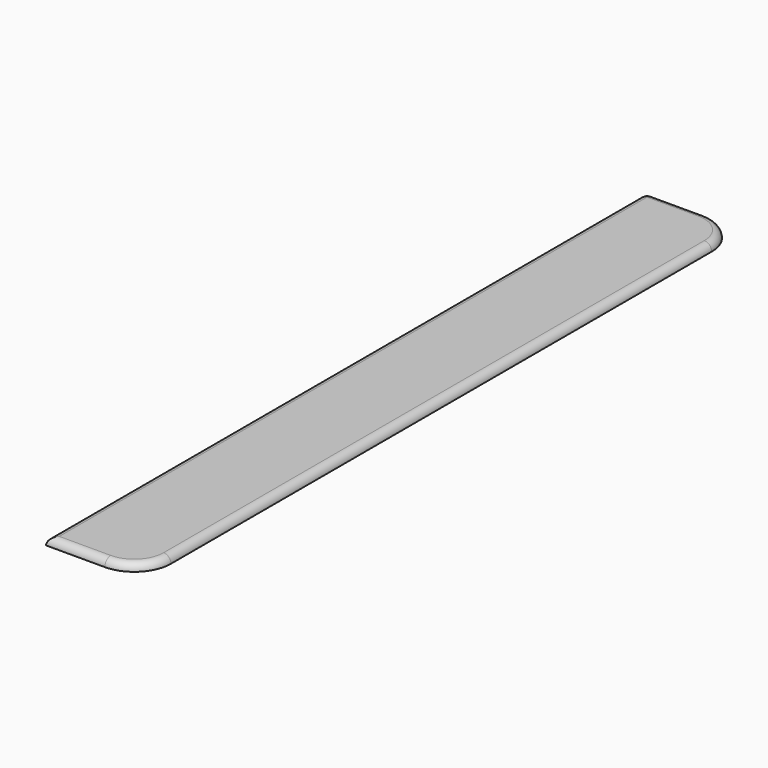
from build123d import *

# Parameters (mm, degrees)
F1_DEPTH     = 1
F2_W         = 1.7
F2_H         = 2
F2_W_2       = 6.3
F2_H_2       = 8
F3_DEPTH     = 1.7
F4_W         = 8
F4_H         = 10
F5_DEPTH     = 2
F6_R         = 5
F7_R         = 0.99999
F8_T1_DEPTH  = 3.7
F8_T3_DEPTH  = 7.5
F8_T5_DEPTH  = 9.5
F8_T7_DEPTH  = 5.5
F8_T9_DEPTH  = 11.5
F8_T12_ANGLE = 90
F8_S15_W     = 1
F8_S15_H     = 1
F8_T16_DEPTH = 1
F8_T20_ANGLE = 90
F10_DEPTH    = 1.7


# Not quite as in the source:
# - a fillet or chamfer that OpenCascade refuses, or shapes differently, is made with other operations: its cross-section is extruded or revolved along the edge and cut away or added
# - a fillet or chamfer is up to 0.001 mm smaller than in the source, because OpenCascade refuses the exact size


with BuildPart() as f1:
    # F0 (on Top) → F1 (new body)
    with BuildSketch(Plane.XY):
        with BuildLine():
            Line((-6.5, -51), (6.5, -51))
            Line((6.5, -51), (6.5, 46))
            ThreePointArc((6.5, 46), (5.0355339059, 49.5355339059), (1.5, 51))
            Line((1.5, 51), (-6.5, 51))
            Line((-6.5, 51), (-6.5, -51))
        make_face()
    extrude(amount=F1_DEPTH)

    # F2 (on face) → F3 (join)
    with BuildSketch(Plane(origin=(0, 0, 0), x_dir=(1, 0, 0), z_dir=(0, 0, -1))):
        with Locations((-5.65, -50)):
            Rectangle(F2_W, F2_H)
        with Locations((-1.65, -50)):
            Rectangle(F2_W_2, F2_H)
        with Locations((-5.65, -45)):
            Rectangle(F2_W, F2_H_2)
    extrude(amount=F3_DEPTH)

    # F4 (on face) → F5 (join)
    with BuildSketch(Plane(origin=(0, 0, -1.7), x_dir=(1, 0, 0), z_dir=(0, 0, -1))):
        with Locations((-2.5, -46)):
            Rectangle(F4_W, F4_H)
    extrude(amount=F5_DEPTH)

    # F6
    f6_edges = [f1.edges().sort_by_distance(p)[0] for p in [
        (6.5, -51, 0.5),
        (1.5, 41, -2.7),
    ]]
    fillet(f6_edges, radius=F6_R)

    # F7 (radius 1 in the source; OpenCascade refuses exactly that, so slightly less here)
    f7_edges = [f1.edges().sort_by_distance(p)[0] for p in [
        (-2.5, -51, 1),
        (5.035534, -49.535534, 1),
        (-6.5, 0, 1),
        (6.5, 0, 1),
        (-2.5, 51, 1),
        (5.035534, 49.535534, 1),
    ]]
    fillet(f7_edges, radius=F7_R)

    # F8: fillet of radius 1 on 6 edges, made by hand

    # F8_s2 → F8_t1 (cut)
    with BuildSketch(Plane.XY.offset(-2.7)):
        with BuildLine():
            ThreePointArc((-5.5, 51), (-6.2071067812, 50.7071067812), (-6.5, 50))
            Line((-6.5, 50), (-6.5, 51))
            Line((-6.5, 51), (-5.5, 51))
        make_face()
    extrude(amount=F8_T1_DEPTH, mode=Mode.SUBTRACT)

    # F8_s4 → F8_t3 (cut)
    with BuildSketch(Plane.XZ.offset(-53.5)):
        with BuildLine():
            ThreePointArc((1.5, -2.7), (1.2071067812, -3.4071067812), (0.5, -3.7))
            Line((0.5, -3.7), (1.5, -3.7))
            Line((1.5, -3.7), (1.5, -2.7))
        make_face()
    extrude(amount=F8_T3_DEPTH, mode=Mode.SUBTRACT)

    # F8_s6 → F8_t5 (cut)
    with BuildSketch(Plane.YZ.offset(-5.5)):
        with BuildLine():
            ThreePointArc((51, -2.7), (50.7071067812, -3.4071067812), (50, -3.7))
            Line((50, -3.7), (51, -3.7))
            Line((51, -3.7), (51, -2.7))
        make_face()
    extrude(amount=F8_T5_DEPTH, mode=Mode.SUBTRACT)

    # F8_s8 → F8_t7 (cut)
    with BuildSketch(Plane.YZ.offset(-9)):
        with BuildLine():
            ThreePointArc((42, -3.7), (41.2928932188, -3.4071067812), (41, -2.7))
            Line((41, -2.7), (41, -3.7))
            Line((41, -3.7), (42, -3.7))
        make_face()
    extrude(amount=F8_T7_DEPTH, mode=Mode.SUBTRACT)

    # F8_s10 → F8_t9 (cut)
    with BuildSketch(Plane.XZ.offset(-50)):
        with BuildLine():
            ThreePointArc((-6.5, -2.7), (-6.2071067812, -3.4071067812), (-5.5, -3.7))
            Line((-5.5, -3.7), (-6.5, -3.7))
            Line((-6.5, -3.7), (-6.5, -2.7))
        make_face()
    extrude(amount=F8_T9_DEPTH, mode=Mode.SUBTRACT)

    # F8_s11 → F8_t12 (revolve, cut)
    with BuildSketch(Plane.YZ.offset(-5.5)):
        with BuildLine():
            ThreePointArc((50.00001, 1), (50.7071097101, 0.7071097101), (51, 1e-05))
            Line((51, 1e-05), (51, 1))
            Line((51, 1), (50.00001, 1))
        make_face()
    revolve(axis=Axis((-5.5, 50, 1), (0, 0, 1)), revolution_arc=F8_T12_ANGLE, mode=Mode.SUBTRACT)


with BuildPart() as f8_tool14:
    # F8_s15 → F8_t16 (new body)
    with BuildSketch(Plane.XZ.offset(-50)):
        with Locations((-6, -3.2)):
            Rectangle(F8_S15_W, F8_S15_H)
    extrude(amount=-F8_T16_DEPTH)

    # F8_s17 → F8_t18 (revolve, cut)
    with BuildSketch(Plane(origin=(-5.5, 50, -2.7), x_dir=(0.7071067812, 0, 0.7071067812), z_dir=(-0.7071067812, 0, 0.7071067812))):
        with BuildLine():
            ThreePointArc((0, -1), (1, 0), (0, 1))
            Line((0, 1), (0, -1))
        make_face()
    revolve(axis=Axis((-5.5, 50, -2.7), (0, 1, 0)), mode=Mode.SUBTRACT)


with BuildPart() as f1_1:
    add(f1.part)

    # F8_t13: cut F8_tool14
    add(f8_tool14.part, mode=Mode.SUBTRACT)

    # F8_s19 → F8_t20 (revolve, cut)
    with BuildSketch(Plane.XZ.offset(-46)):
        with BuildLine():
            ThreePointArc((0.5, -3.7), (1.2071067812, -3.4071067812), (1.5, -2.7))
            Line((1.5, -2.7), (1.5, -3.7))
            Line((1.5, -3.7), (0.5, -3.7))
        make_face()
    revolve(axis=Axis((-3.5, 46, -3.7), (0, 0, -1)), revolution_arc=F8_T20_ANGLE, mode=Mode.SUBTRACT)

    # F9 (on face) → F10 (join, through all)
    with BuildSketch(Plane(origin=(0, 0, 0), x_dir=(1, 0, 0), z_dir=(0, 0, -1))):
        with BuildLine():
            ThreePointArc((-3.5, -42), (-0.6715728753, -43.1715728753), (0.5, -46))
            Line((0.5, -46), (1.5, -46))
            ThreePointArc((1.5, -46), (0.0355339059, -42.4644660941), (-3.5, -41))
            Line((-3.5, -41), (-3.5, -42))
        make_face()
    extrude(amount=F10_DEPTH)


solid = f1_1.part
